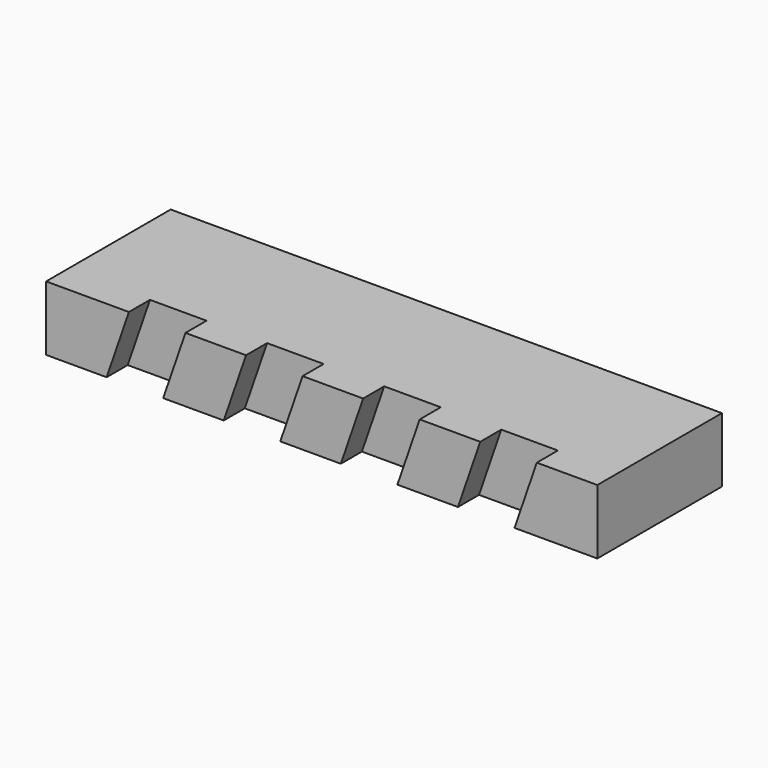
from build123d import *

# Parameters (mm, degrees)
F1_DEPTH = 10
F2_SIZE2 = 3.442485
F2_SIZE  = 9.99999
F3_SIZE2 = 3.442485
F3_SIZE  = 9.99999
F4_SIZE2 = 3.442485
F4_SIZE  = 9.99999
F5_SIZE2 = 3.442485
F5_SIZE  = 9.99999
F6_SIZE2 = 3.442485
F6_SIZE  = 9.99999
F7_SIZE2 = 3.442485
F7_SIZE  = 9.99999
F8_SIZE2 = 3.442485
F8_SIZE  = 9.99999
F9_SIZE2 = 3.442485
F9_SIZE  = 9.99999


# Not quite as in the source:
# - a fillet or chamfer is up to 0.001 mm smaller than in the source, because OpenCascade refuses the exact size


with BuildPart() as f1:
    # F0 (on Top) → F1 (new body)
    with BuildSketch(Plane.XY):
        Polygon((41.1003320895, 9.3217377585), (-44.0996679105, 9.3217377585), (-44.0996679105, -10.6782622415), (-44.0996679105, -14.7482622415), (-31.2996679105, -14.7482622415), (-31.2996679105, -10.6782622415), (-25.9996679105, -10.6782622415), (-25.9996679105, -14.7482622415), (-13.1996679105, -14.7482622415), (-13.1996679105, -10.6782622415), (-7.8996679105, -10.6782622415), (-7.8996679105, -14.7482622415), (4.9003320895, -14.7482622415), (4.9003320895, -10.6782622415), (10.2003320895, -10.6782622415), (10.2003320895, -14.7482622415), (23.0003320895, -14.7482622415), (23.0003320895, -10.6782622415), (28.3003320895, -10.6782622415), (28.3003320895, -14.7482622415), (41.1003320895, -14.7482622415), (41.1003320895, -10.6782622415), align=None)
    extrude(amount=F1_DEPTH)

    # F2 (size 10 and 3.4424952484 in the source; OpenCascade refuses exactly that, so slightly less here)
    f2_edges = [f1.edges().sort_by_distance(p)[0] for p in [
        (-31.299668, -12.713262, 0),
    ]]
    f2_side = f1.faces().sort_by_distance((-31.299668, -12.713262, 5))[0]
    chamfer(f2_edges, length=F2_SIZE, length2=F2_SIZE2, reference=f2_side)

    # F3 (size 10 and 3.4424952484 in the source; OpenCascade refuses exactly that, so slightly less here)
    f3_edges = [f1.edges().sort_by_distance(p)[0] for p in [
        (-25.999668, -12.713262, 10),
    ]]
    f3_side = f1.faces().sort_by_distance((-25.999668, -12.713262, 5))[0]
    chamfer(f3_edges, length=F3_SIZE, length2=F3_SIZE2, reference=f3_side)

    # F4 (size 10 and 3.4424952484 in the source; OpenCascade refuses exactly that, so slightly less here)
    f4_edges = [f1.edges().sort_by_distance(p)[0] for p in [
        (-13.199668, -12.713262, 0),
    ]]
    f4_side = f1.faces().sort_by_distance((-13.199668, -12.713262, 5))[0]
    chamfer(f4_edges, length=F4_SIZE, length2=F4_SIZE2, reference=f4_side)

    # F5 (size 10 and 3.4424952484 in the source; OpenCascade refuses exactly that, so slightly less here)
    f5_edges = [f1.edges().sort_by_distance(p)[0] for p in [
        (-7.899668, -12.713262, 10),
    ]]
    f5_side = f1.faces().sort_by_distance((-7.899668, -12.713262, 5))[0]
    chamfer(f5_edges, length=F5_SIZE, length2=F5_SIZE2, reference=f5_side)

    # F6 (size 10 and 3.4424952484 in the source; OpenCascade refuses exactly that, so slightly less here)
    f6_edges = [f1.edges().sort_by_distance(p)[0] for p in [
        (4.900332, -12.713262, 0),
    ]]
    f6_side = f1.faces().sort_by_distance((4.900332, -12.713262, 5))[0]
    chamfer(f6_edges, length=F6_SIZE, length2=F6_SIZE2, reference=f6_side)

    # F7 (size 10 and 3.4424952484 in the source; OpenCascade refuses exactly that, so slightly less here)
    f7_edges = [f1.edges().sort_by_distance(p)[0] for p in [
        (10.200332, -12.713262, 10),
    ]]
    f7_side = f1.faces().sort_by_distance((10.200332, -12.713262, 5))[0]
    chamfer(f7_edges, length=F7_SIZE, length2=F7_SIZE2, reference=f7_side)

    # F8 (size 10 and 3.4424952484 in the source; OpenCascade refuses exactly that, so slightly less here)
    f8_edges = [f1.edges().sort_by_distance(p)[0] for p in [
        (23.000332, -12.713262, 0),
    ]]
    f8_side = f1.faces().sort_by_distance((23.000332, -12.713262, 5))[0]
    chamfer(f8_edges, length=F8_SIZE, length2=F8_SIZE2, reference=f8_side)

    # F9 (size 10 and 3.4424952484 in the source; OpenCascade refuses exactly that, so slightly less here)
    f9_edges = [f1.edges().sort_by_distance(p)[0] for p in [
        (28.300332, -12.713262, 10),
    ]]
    f9_side = f1.faces().sort_by_distance((28.300332, -12.713262, 5))[0]
    chamfer(f9_edges, length=F9_SIZE, length2=F9_SIZE2, reference=f9_side)


solid = f1.part
